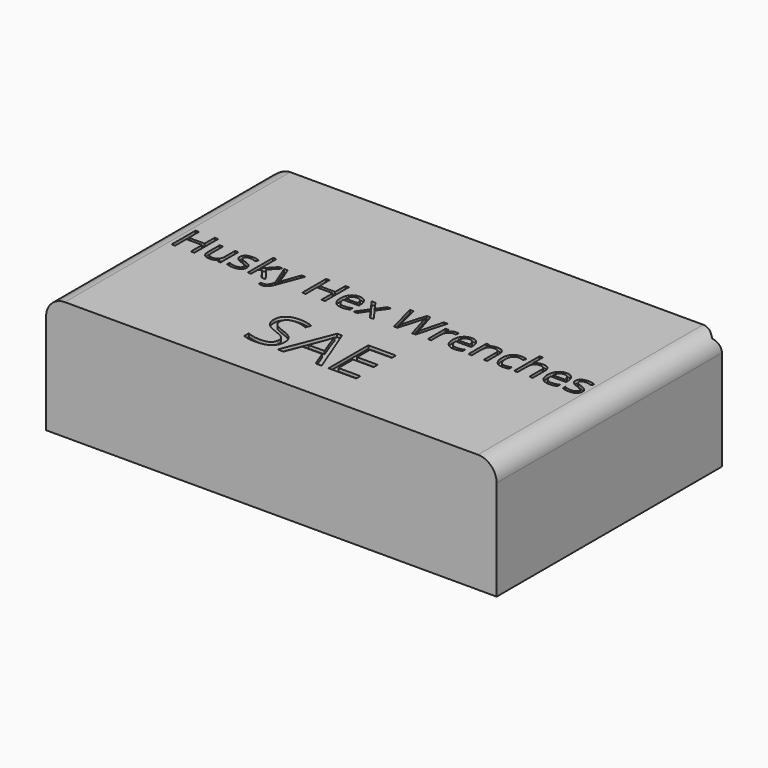
from build123d import *

# Parameters (mm, degrees)
F0_W           = 72
F0_H           = 19
F0_W_2         = 66
F0_H_2         = 13
F1_DEPTH       = 22.5
F2_R           = 3
F3_T1_DEPTH    = 66
F3_T3_DEPTH    = 13
F3_T9_DEPTH    = 20.7150489639
F3_T14_DEPTH   = 73.7150489639
F3_T22_DEPTH   = 73.7150489639
F3_T27_DEPTH   = 20.7150489639
F3_T35_DEPTH   = 20.7150489639
F3_S36_R       = 3
F3_T37_DEPTH   = 12
F3_T41_DEPTH   = 73.7150489639
F3_S42_R       = 3
F3_T43_DEPTH   = 38
F3_T50_DEPTH   = 20.7150489639
F3_S51_R       = 3
F3_T52_DEPTH   = 12
F3_T56_DEPTH   = 73.7150489639
F3_S57_R       = 3
F3_T58_DEPTH   = 38
F5_W           = 66
F5_H           = 13
F6_DEPTH       = 1
F7_TEXT_SIZE   = 6.6966833661
F7_TEXT_SIZE_2 = 11.1239535424
F8_DEPTH       = 0.5


# Not quite as in the source:
# - a fillet or chamfer that OpenCascade refuses, or shapes differently, is made with other operations: its cross-section is extruded or revolved along the edge and cut away or added
# - Text() gives the source's letters only with a copy of the font that has no kerning and outlines rounded to 1/6400 em; it was checked with that copy


with BuildPart() as f1:
    # F0 (on Front) → F1 (new body, symmetric)
    with BuildSketch(Plane.XZ):
        Rectangle(F0_W, F0_H)
        Rectangle(F0_W_2, F0_H_2, mode=Mode.SUBTRACT)
    extrude(amount=F1_DEPTH, both=True)

    # F2
    f2_edges = [f1.edges().sort_by_distance(p)[0] for p in [
        (-36, 0, 9.5),
        (36, 0, 9.5),
    ]]
    fillet(f2_edges, radius=F2_R)

    # F3: chamfer of 3 on 4 edges, made by hand

    # F3_s2 → F3_t1 (cut)
    with BuildSketch(Plane.YZ.offset(-33)):
        Polygon((22.5, -9.5), (19.5, -6.5), (22.5, -6.5), align=None)
        Polygon((22.5, 9.5), (19.5, 6.5), (22.5, 6.5), align=None)
    extrude(amount=F3_T1_DEPTH, mode=Mode.SUBTRACT)

    # F3_s4 → F3_t3 (cut)
    with BuildSketch(Plane.XY.offset(-6.5)):
        Polygon((36, 22.5), (33, 19.5), (33, 22.5), align=None)
        Polygon((-36, 22.5), (-33, 19.5), (-33, 22.5), align=None)
    extrude(amount=F3_T3_DEPTH, mode=Mode.SUBTRACT)


with BuildPart() as f3_tool7:
    # F3_s8 → F3_t9 (new body)
    with BuildSketch(Plane.XY.offset(6.5)):
        Polygon((36, 22.5), (33, 19.5), (33, 22.5), align=None)
    extrude(amount=-F3_T9_DEPTH)

    split(bisect_by=Plane.XY.offset(-9.5), keep=Keep.TOP)

    split(bisect_by=Plane.XY.offset(-6.5), keep=Keep.BOTTOM)


with BuildPart() as f3_tool12:
    # F3_s13 → F3_t14 (new body)
    with BuildSketch(Plane.YZ.offset(40.7150489639)):
        Polygon((22.5, -9.5), (19.5, -6.5), (22.5, -6.5), align=None)
    extrude(amount=-F3_T14_DEPTH)

    split(bisect_by=Plane.YZ.offset(36), keep=Keep.BOTTOM)

    split(bisect_by=Plane.YZ.offset(33), keep=Keep.TOP)


with BuildPart() as f3_tool7_1:
    add(f3_tool7.part)

    # F3_t17: intersect F3_tool12
    add(f3_tool12.part, mode=Mode.INTERSECT)


with BuildPart() as f1_1:
    add(f1.part)

    # F3_t5: cut F3_tool7
    add(f3_tool7_1.part, mode=Mode.SUBTRACT)


with BuildPart() as f3_tool20:
    # F3_s21 → F3_t22 (new body)
    with BuildSketch(Plane.YZ.offset(33)):
        Polygon((22.5, -9.5), (19.5, -6.5), (22.5, -6.5), align=None)
    extrude(amount=-F3_T22_DEPTH)

    split(bisect_by=Plane.YZ.offset(-36), keep=Keep.TOP)

    split(bisect_by=Plane.YZ.offset(-33), keep=Keep.BOTTOM)


with BuildPart() as f3_tool25:
    # F3_s26 → F3_t27 (new body)
    with BuildSketch(Plane.XY.offset(-14.2150489639)):
        Polygon((-36, 22.5), (-33, 19.5), (-33, 22.5), align=None)
    extrude(amount=F3_T27_DEPTH)

    split(bisect_by=Plane.XY.offset(-9.5), keep=Keep.TOP)

    split(bisect_by=Plane.XY.offset(-6.5), keep=Keep.BOTTOM)


with BuildPart() as f3_tool20_1:
    add(f3_tool20.part)

    # F3_t30: intersect F3_tool25
    add(f3_tool25.part, mode=Mode.INTERSECT)


with BuildPart() as f1_2:
    add(f1_1.part)

    # F3_t18: cut F3_tool20
    add(f3_tool20_1.part, mode=Mode.SUBTRACT)


with BuildPart() as f3_tool33:
    # F3_s34 → F3_t35 (new body)
    with BuildSketch(Plane.XY.offset(-6.5)):
        Polygon((-36, 22.5), (-33, 19.5), (-33, 22.5), align=None)
    extrude(amount=F3_T35_DEPTH)

    # F3_s36 → F3_t37 (intersect, symmetric)
    with BuildSketch(Plane.XZ.offset(-21)):
        with Locations((-33, 6.5)):
            Circle(F3_S36_R)
    extrude(amount=F3_T37_DEPTH, both=True, mode=Mode.INTERSECT)

    split(bisect_by=Plane.XY.offset(6.5), keep=Keep.TOP)


with BuildPart() as f3_tool39:
    # F3_s40 → F3_t41 (new body)
    with BuildSketch(Plane.YZ.offset(-40.7150489639)):
        Polygon((22.5, 9.5), (19.5, 6.5), (22.5, 6.5), align=None)
    extrude(amount=F3_T41_DEPTH)

    # F3_s42 → F3_t43 (intersect, symmetric)
    with BuildSketch(Plane.XZ.offset(-21)):
        with Locations((-33, 6.5)):
            Circle(F3_S42_R)
    extrude(amount=F3_T43_DEPTH, both=True, mode=Mode.INTERSECT)

    split(bisect_by=Plane.YZ.offset(-33), keep=Keep.BOTTOM)


with BuildPart() as f3_tool33_1:
    add(f3_tool33.part)

    # F3_t45: intersect F3_tool39
    add(f3_tool39.part, mode=Mode.INTERSECT)


with BuildPart() as f1_3:
    add(f1_2.part)

    # F3_t31: cut F3_tool33
    add(f3_tool33_1.part, mode=Mode.SUBTRACT)


with BuildPart() as f3_tool48:
    # F3_s49 → F3_t50 (new body)
    with BuildSketch(Plane.XY.offset(14.2150489639)):
        Polygon((36, 22.5), (33, 19.5), (33, 22.5), align=None)
    extrude(amount=-F3_T50_DEPTH)

    # F3_s51 → F3_t52 (intersect, symmetric)
    with BuildSketch(Plane.XZ.offset(-21)):
        with Locations((33, 6.5)):
            Circle(F3_S51_R)
    extrude(amount=F3_T52_DEPTH, both=True, mode=Mode.INTERSECT)

    split(bisect_by=Plane.XY.offset(6.5), keep=Keep.TOP)


with BuildPart() as f3_tool54:
    # F3_s55 → F3_t56 (new body)
    with BuildSketch(Plane.YZ.offset(-33)):
        Polygon((22.5, 9.5), (19.5, 6.5), (22.5, 6.5), align=None)
    extrude(amount=F3_T56_DEPTH)

    # F3_s57 → F3_t58 (intersect, symmetric)
    with BuildSketch(Plane.XZ.offset(-21)):
        with Locations((33, 6.5)):
            Circle(F3_S57_R)
    extrude(amount=F3_T58_DEPTH, both=True, mode=Mode.INTERSECT)

    split(bisect_by=Plane.YZ.offset(33), keep=Keep.TOP)


with BuildPart() as f3_tool48_1:
    add(f3_tool48.part)

    # F3_t60: intersect F3_tool54
    add(f3_tool54.part, mode=Mode.INTERSECT)


with BuildPart() as f1_4:
    add(f1_3.part)

    # F3_t46: cut F3_tool48
    add(f3_tool48_1.part, mode=Mode.SUBTRACT)

    # F5 (on face) → F6 (join)
    with BuildSketch(Plane.XZ.offset(22.5)):
        Rectangle(F5_W, F5_H)
    extrude(amount=-F6_DEPTH)

    # F7 (on face) → F8 (cut, symmetric)
    with BuildSketch(Plane.XY.offset(9.5)):
        with Locations((-33, -2.0017799266)):
            Text('Husky Hex Wrenches', F7_TEXT_SIZE, font='Open Sans', text_align=(TextAlign.LEFT, TextAlign.BOTTOM))
        with Locations((-10.381501168, -15.9004572779)):
            Text('SAE', F7_TEXT_SIZE_2, font='Open Sans', text_align=(TextAlign.LEFT, TextAlign.BOTTOM))
    extrude(amount=F8_DEPTH, both=True, mode=Mode.SUBTRACT)


solid = f1_4.part
